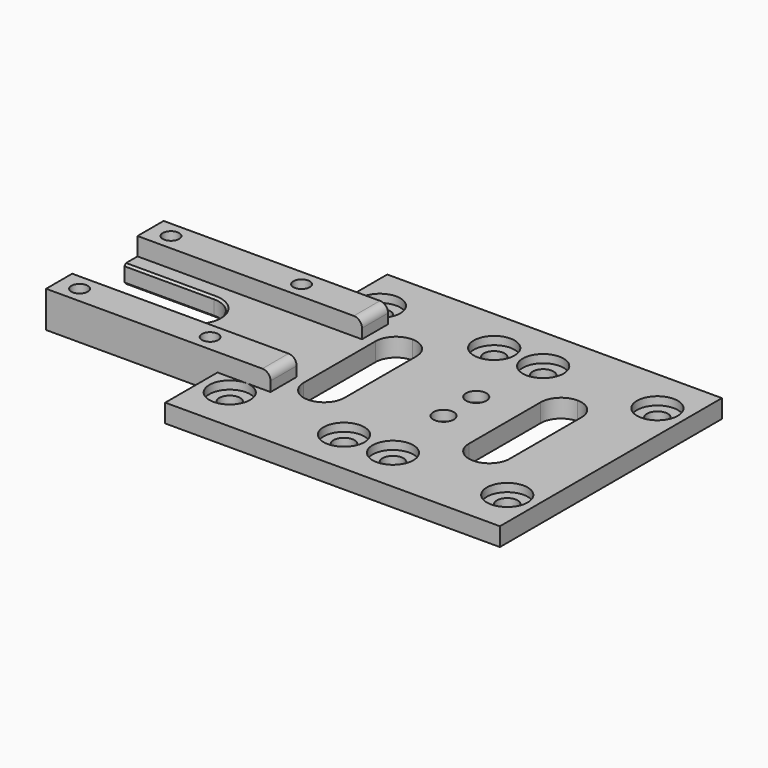
from build123d import *

# Parameters (mm, degrees)
F1_DEPTH  = 4.5
F2_R      = 2.55
F3_DEPTH  = 25
F4_W      = 55
F4_H      = 8
F5_DEPTH  = 4.4
F6_R      = 2.5
F7_DEPTH  = 25
F8_R      = 2
F9_DEPTH  = 25
F10_W     = 10
F10_H     = 32
F11_DEPTH = 25
F12_R     = 4.99999
F13_R     = 4.99999
F14_R     = 2
F15_R     = 5
F16_DEPTH = 2
F18_DEPTH = 2
F19_SIZE  = 0.5
F20_SIZE  = 0.5
F21_DEPTH = 25


# Not quite as in the source:
# - a fillet or chamfer is up to 0.001 mm smaller than in the source, because OpenCascade refuses the exact size


with BuildPart() as f1:
    # F0 (on Top) → F1 (new body)
    with BuildSketch(Plane.XY):
        with BuildLine():
            Line((0, 16), (0, 0))
            Line((0, 0), (82, 0))
            Line((82, 0), (82, 68))
            Line((82, 68), (0, 68))
            Line((0, 68), (0, 52))
            Line((0, 52), (-42, 52))
            Line((-42, 52), (-42, 40))
            Line((-42, 40), (-20.0227203867, 40))
            ThreePointArc((-20.0227203867, 40), (-14.0227203867, 34), (-20.0227203867, 28))
            Line((-20.0227203867, 28), (-42, 28))
            Line((-42, 28), (-42, 16))
            Line((-42, 16), (0, 16))
        make_face()
    extrude(amount=F1_DEPTH)

    # F2 (on face) → F3 (cut)
    with BuildSketch(Plane.XY.offset(4.5)):
        with Locations((75, 57)):
            Circle(F2_R)
        with Locations((75, 11)):
            Circle(F2_R)
        with Locations((47, 57)):
            Circle(F2_R)
        with Locations((47, 11)):
            Circle(F2_R)
        with Locations((35, 57)):
            Circle(F2_R)
        with Locations((35, 11)):
            Circle(F2_R)
        with Locations((7, 57)):
            Circle(F2_R)
        with Locations((7, 11)):
            Circle(F2_R)
    extrude(amount=-F3_DEPTH, mode=Mode.SUBTRACT)

    # F4 (on face) → F5 (join)
    with BuildSketch(Plane.XY.offset(4.5)):
        with Locations((-14.5, 48)):
            Rectangle(F4_W, F4_H)
        with Locations((-14.5, 20)):
            Rectangle(F4_W, F4_H)
    extrude(amount=F5_DEPTH)

    # F6 (on face) → F7 (cut)
    with BuildSketch(Plane.XY.offset(4.5)):
        with Locations((45, 29)):
            Circle(F6_R)
        with Locations((45, 39)):
            Circle(F6_R)
    extrude(amount=-F7_DEPTH, mode=Mode.SUBTRACT)

    # F8 (on face) → F9 (cut)
    with BuildSketch(Plane(origin=(0, 0, 0), x_dir=(1, 0, 0), z_dir=(0, 0, -1))):
        with Locations((-37, -48)):
            Circle(F8_R)
        with Locations((-5, -48)):
            Circle(F8_R)
        with Locations((-37, -20)):
            Circle(F8_R)
        with Locations((-5, -20)):
            Circle(F8_R)
    extrude(amount=-F9_DEPTH, mode=Mode.SUBTRACT)

    # F10 (on face) → F11 (cut)
    with BuildSketch(Plane.XY.offset(4.5)):
        with Locations((61, 34)):
            Rectangle(F10_W, F10_H)
        with Locations((20.5358764028, 34)):
            Rectangle(F10_W, F10_H)
    extrude(amount=-F11_DEPTH, mode=Mode.SUBTRACT)

    # F12 (radius 5 in the source; OpenCascade refuses exactly that, so slightly less here)
    f12_edges = [f1.edges().sort_by_distance(p)[0] for p in [
        (15.535876, 50, 2.25),
        (25.535876, 50, 2.25),
        (15.535876, 18, 2.25),
        (25.535876, 18, 2.25),
    ]]
    fillet(f12_edges, radius=F12_R)

    # F13 (radius 5 in the source; OpenCascade refuses exactly that, so slightly less here)
    f13_edges = [f1.edges().sort_by_distance(p)[0] for p in [
        (56, 18, 2.25),
        (66, 18, 2.25),
        (66, 50, 2.25),
        (56, 50, 2.25),
    ]]
    fillet(f13_edges, radius=F13_R)

    # F14
    f14_edges = [f1.edges().sort_by_distance(p)[0] for p in [
        (13, 48, 8.9),
        (13, 20, 8.9),
    ]]
    fillet(f14_edges, radius=F14_R)

    # F15 (on face) → F16 (cut)
    with BuildSketch(Plane.XY.offset(4.5)):
        with Locations((75, 11)):
            Circle(F15_R)
        with Locations((47, 11)):
            Circle(F15_R)
        with Locations((35, 11)):
            Circle(F15_R)
        with Locations((7, 11)):
            Circle(F15_R)
        with Locations((7, 57)):
            Circle(F15_R)
        with Locations((35, 57)):
            Circle(F15_R)
        with Locations((47, 57)):
            Circle(F15_R)
        with Locations((75, 57)):
            Circle(F15_R)
    extrude(amount=-F16_DEPTH, mode=Mode.SUBTRACT)

    # F17 (on face) → F18 (cut)
    with BuildSketch(Plane(origin=(0, 0, 0), x_dir=(1, 0, 0), z_dir=(0, 0, -1))):
        with BuildLine():
            Line((40.0007831694, -39.0884933935), (40.0007694899, -38.9122828006))
            ThreePointArc((40.0007694899, -38.9122828006), (40.0000000151, -39.0003881573), (40.0007831694, -39.0884933935))
        make_face()
        with BuildLine():
            Line((40.0000000151, -29.0003881573), (40.0007694899, -38.9122828006))
            Line((40.0007694899, -38.9122828006), (40.0007831694, -39.0884933935))
            ThreePointArc((40.0007831694, -39.0884933935), (45.0442484332, -43.9998042038), (50, -38.9999999925))
            Line((50, -38.9999999925), (49.9999999849, -29.0003881573))
            ThreePointArc((49.9999999849, -29.0003881573), (45, -24), (40.0000000151, -29.0003881573))
        make_face()
    extrude(amount=-F18_DEPTH, mode=Mode.SUBTRACT)

    # F19
    f19_edges = [f1.edges().sort_by_distance(p)[0] for p in [
        (-31.01136, 28, 4.5),
        (-31.01136, 40, 4.5),
        (-14.02272, 34, 4.5),
    ]]
    chamfer(f19_edges, length=F19_SIZE)

    # F20
    f20_edges = [f1.edges().sort_by_distance(p)[0] for p in [
        (-31.01136, 40, 0),
        (-31.01136, 28, 0),
        (-14.02272, 34, 0),
    ]]
    chamfer(f20_edges, length=F20_SIZE)

    # F8 (on face) → F21 (cut)
    with BuildSketch(Plane(origin=(0, 0, 0), x_dir=(1, 0, 0), z_dir=(0, 0, -1))):
        with Locations((-37, -48)):
            Circle(F8_R)
        with Locations((-5, -48)):
            Circle(F8_R)
        with Locations((-37, -20)):
            Circle(F8_R)
        with Locations((-5, -20)):
            Circle(F8_R)
    extrude(amount=-F21_DEPTH, mode=Mode.SUBTRACT)


solid = f1.part
